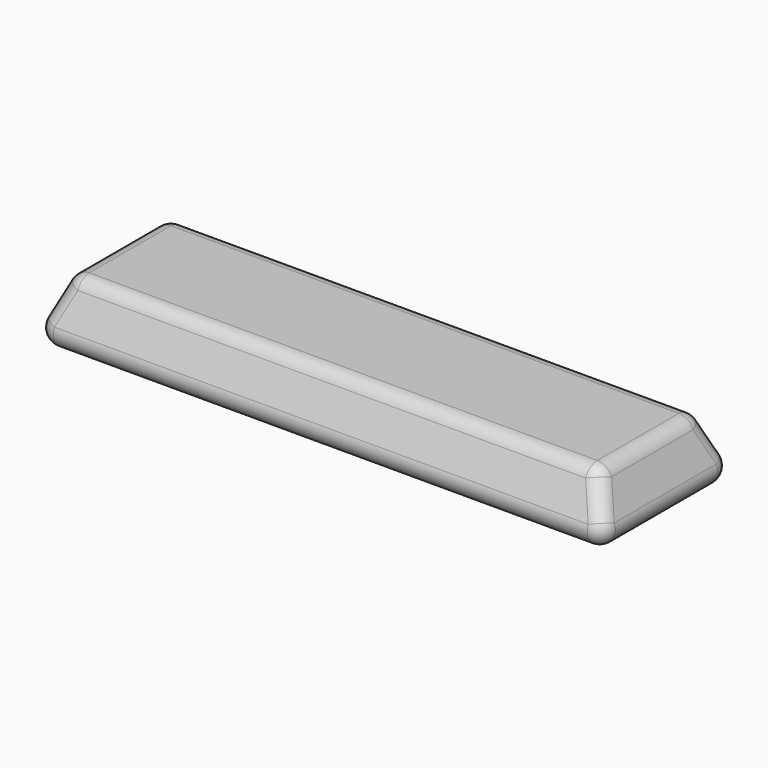
from build123d import *

# Parameters (mm, degrees)
F0_W         = 240
F0_H         = 110
F1_DEPTH     = 20
F2_T1_DEPTH  = 499.2670392907
F3_T1_DEPTH  = 865.9260025319
F4_T1_DEPTH  = 298.556361172
F5_T1_DEPTH  = 665.2153244132
F6_R         = 5
F7_T1_DEPTH  = 170.8918067496
F7_T3_DEPTH  = 40.8918067496
F7_S7_W      = 28.0904022212
F7_S7_H      = 28.0904022212
F7_T8_DEPTH  = 14.0452011106
F7_S19_W     = 28.0904022212
F7_S19_H     = 28.0904022211
F7_T20_DEPTH = 14.0452011106
F7_S31_W     = 28.0904022212
F7_S31_H     = 28.0904022212
F7_T32_DEPTH = 14.0452011106
F7_S43_W     = 28.0904022212
F7_S43_H     = 28.0904022212
F7_T44_DEPTH = 14.0452011106


# Not quite as in the source:
# - a fillet or chamfer that OpenCascade refuses, or shapes differently, is made with other operations: its cross-section is extruded or revolved along the edge and cut away or added


with BuildPart() as f1:
    # F0 (on Top) → F1 (new body)
    with BuildSketch(Plane.XY):
        Rectangle(F0_W, F0_H)
    extrude(amount=F1_DEPTH)

    # F2: chamfer of 50 x 20.7106781187 on 1 edges, made by hand

    # F2_s2 → F2_t1 (cut)
    with BuildSketch(Plane.YZ.offset(-249.6335196453)):
        Polygon((-55, -30), (-34.2893218813, 20), (-55, 20), align=None)
    extrude(amount=F2_T1_DEPTH, mode=Mode.SUBTRACT)

    # F3: chamfer of 50 x 120.7106781187 on 1 edges, made by hand

    # F3_s2 → F3_t1 (cut)
    with BuildSketch(Plane.YZ.offset(-432.9630012659)):
        Polygon((55, -100.7106781187), (5, 20), (55, 20), align=None)
    extrude(amount=F3_T1_DEPTH, mode=Mode.SUBTRACT)

    # F4: chamfer of 50 x 20.7106781187 on 1 edges, made by hand

    # F4_s2 → F4_t1 (cut)
    with BuildSketch(Plane.XZ.offset(-134.6335196453)):
        Polygon((120, -30), (99.2893218813, 20), (120, 20), align=None)
    extrude(amount=F4_T1_DEPTH, mode=Mode.SUBTRACT)

    # F5: chamfer of 50 x 120.7106781187 on 1 edges, made by hand

    # F5_s2 → F5_t1 (cut)
    with BuildSketch(Plane.XZ.offset(-317.9630012659)):
        Polygon((-120, -100.7106781187), (-70, 20), (-120, 20), align=None)
    extrude(amount=F5_T1_DEPTH, mode=Mode.SUBTRACT)

    # F6
    f6_edges = [f1.edges().sort_by_distance(p)[0] for p in [
        (103.431458, -38.431458, 10),
        (99.289322, -14.644661, 20),
        (14.644661, -34.289322, 20),
        (-74.142136, -38.431458, 10),
        (-70, -14.644661, 20),
        (-74.142136, 9.142136, 10),
        (103.431458, 9.142136, 10),
        (14.644661, 5, 20),
    ]]
    fillet(f6_edges, radius=F6_R)

    # F7: fillet of radius 5 on 8 edges, made by hand

    # F7_s2 → F7_t1 (cut)
    with BuildSketch(Plane.YZ.offset(-70.8012424341)):
        with BuildLine():
            ThreePointArc((5.8012424341, 0), (9.9585904956, 2.2221488349), (10.4206400967, 6.9134171618))
            Line((10.4206400967, 6.9134171618), (13.2842712475, 0))
            Line((13.2842712475, 0), (5.8012424341, 0))
        make_face()
        with BuildLine():
            ThreePointArc((-35.0905643154, 0), (-39.247912377, 2.2221488349), (-39.709961978, 6.9134171618))
            Line((-39.709961978, 6.9134171618), (-42.5735931288, 0))
            Line((-42.5735931288, 0), (-35.0905643154, 0))
        make_face()
    extrude(amount=F7_T1_DEPTH, mode=Mode.SUBTRACT)

    # F7_s4 → F7_t3 (cut)
    with BuildSketch(Plane.XZ.offset(-5.8012424341)):
        with BuildLine():
            ThreePointArc((-70.8012424341, 0), (-74.9585904956, 2.2221488349), (-75.4206400967, 6.9134171618))
            Line((-75.4206400967, 6.9134171618), (-78.2842712475, 0))
            Line((-78.2842712475, 0), (-70.8012424341, 0))
        make_face()
        with BuildLine():
            ThreePointArc((100.0905643154, 0), (104.247912377, 2.2221488349), (104.709961978, 6.9134171618))
            Line((104.709961978, 6.9134171618), (107.5735931288, 0))
            Line((107.5735931288, 0), (100.0905643154, 0))
        make_face()
    extrude(amount=F7_T3_DEPTH, mode=Mode.SUBTRACT)


with BuildPart() as f7_tool6:
    # F7_s7 → F7_t8 (new body)
    with BuildSketch(Plane(origin=(-36.4895727765, 36.4895727765, -9.2670771068), x_dir=(-0.7071067812, -0.7071067812, 0), z_dir=(-0.6959735574, 0.6959735574, -0.1767529771))):
        with Locations((45.9619407771, 14.4953021034)):
            Rectangle(F7_S7_W, F7_S7_H)
    extrude(amount=F7_T8_DEPTH)

    split(bisect_by=Plane.YZ.offset(-70.8012424341), keep=Keep.BOTTOM)

    split(bisect_by=Plane(origin=(-8.2432161695, 8.2432161695, -19.900884274), x_dir=(-0.7071067812, -0.7071067812, 0), z_dir=(-0.3574067443, 0.3574067443, -0.8628562095)), keep=Keep.TOP)

    split(bisect_by=Plane.XZ.offset(-5.8012424341), keep=Keep.BOTTOM)

    split(bisect_by=Plane.XY, keep=Keep.TOP)

    split(bisect_by=Plane(origin=(0, 11.3388347648, 4.6966991411), x_dir=(1, 0, 0), z_dir=(0, -0.9238795325, -0.3826834324)), keep=Keep.TOP)

    split(bisect_by=Plane(origin=(-66.8198051534, 0, 27.6776695297), x_dir=(0, 1, 0), z_dir=(0.9238795325, 0, -0.3826834324)), keep=Keep.TOP)

    # F7_s15 → F7_t16 (revolve, cut)
    with BuildSketch(Plane(origin=(-70.8012424341, 5.8012424341, 5), x_dir=(0.6959735574, -0.6959735574, 0.1767529771), z_dir=(0.1249832287, -0.1249832287, -0.9842552439))):
        with BuildLine():
            ThreePointArc((0, -5), (5, 0), (0, 5))
            Line((0, 5), (0, -5))
        make_face()
    revolve(axis=Axis((-70.8012424341, 5.8012424341, 5), (-0.7071067812, -0.7071067812, 0)), mode=Mode.SUBTRACT)


with BuildPart() as f1_1:
    add(f1.part)

    # F7_t5: cut F7_tool6
    add(f7_tool6.part, mode=Mode.SUBTRACT)


with BuildPart() as f7_tool18:
    # F7_s19 → F7_t20 (new body)
    with BuildSketch(Plane(origin=(50.6767108596, 50.6767108597, -12.8701147019), x_dir=(-0.7071067812, 0.7071067812, 0), z_dir=(0.6959735574, 0.6959735574, -0.1767529771))):
        with Locations((-66.6726188958, 18.1559761181)):
            Rectangle(F7_S19_W, F7_S19_H)
    extrude(amount=F7_T20_DEPTH)

    split(bisect_by=Plane.YZ.offset(100.0905643154), keep=Keep.TOP)

    split(bisect_by=Plane(origin=(11.9846218714, 11.9846218714, -28.9334366618), x_dir=(-0.7071067812, 0.7071067812, 0), z_dir=(0.3574067443, 0.3574067443, -0.8628562095)), keep=Keep.TOP)

    split(bisect_by=Plane.XZ.offset(-5.8012424341), keep=Keep.BOTTOM)

    split(bisect_by=Plane.XY, keep=Keep.TOP)

    split(bisect_by=Plane(origin=(0, 11.3388347648, 4.6966991411), x_dir=(1, 0, 0), z_dir=(0, -0.9238795325, -0.3826834324)), keep=Keep.TOP)

    split(bisect_by=Plane(origin=(91.8198051533, 0, 38.033008589), x_dir=(0, 1, 0), z_dir=(-0.9238795325, 0, -0.3826834324)), keep=Keep.TOP)

    # F7_s27 → F7_t28 (revolve, cut)
    with BuildSketch(Plane(origin=(100.0905643154, 5.8012424341, 5), x_dir=(-0.6959735574, -0.6959735574, 0.1767529771), z_dir=(-0.1249832287, -0.1249832287, -0.9842552439))):
        with BuildLine():
            ThreePointArc((0, -5), (5, 0), (0, 5))
            Line((0, 5), (0, -5))
        make_face()
    revolve(axis=Axis((100.0905643154, 5.8012424341, 5), (-0.7071067812, 0.7071067812, 0)), mode=Mode.SUBTRACT)


with BuildPart() as f1_2:
    add(f1_1.part)

    # F7_t17: cut F7_tool18
    add(f7_tool18.part, mode=Mode.SUBTRACT)


with BuildPart() as f7_tool30:
    # F7_s31 → F7_t32 (new body)
    with BuildSketch(Plane(origin=(-50.6767108597, -50.6767108596, -12.8701147019), x_dir=(0.7071067812, -0.7071067812, 0), z_dir=(-0.6959735574, -0.6959735574, -0.1767529771))):
        with Locations((-25.2512626585, 18.1559761181)):
            Rectangle(F7_S31_W, F7_S31_H)
    extrude(amount=F7_T32_DEPTH)

    split(bisect_by=Plane.YZ.offset(-70.8012424341), keep=Keep.BOTTOM)

    split(bisect_by=Plane(origin=(-11.9846218714, -11.9846218714, -28.9334366618), x_dir=(0.7071067812, -0.7071067812, 0), z_dir=(-0.3574067443, -0.3574067443, -0.8628562095)), keep=Keep.TOP)

    split(bisect_by=Plane.XZ.offset(35.0905643154), keep=Keep.TOP)

    split(bisect_by=Plane.XY, keep=Keep.TOP)

    split(bisect_by=Plane(origin=(0, -36.3388347648, 15.0520382004), x_dir=(1, 0, 0), z_dir=(0, 0.9238795325, -0.3826834324)), keep=Keep.TOP)

    split(bisect_by=Plane(origin=(-66.8198051534, 0, 27.6776695297), x_dir=(0, 1, 0), z_dir=(0.9238795325, 0, -0.3826834324)), keep=Keep.TOP)

    # F7_s39 → F7_t40 (revolve, cut)
    with BuildSketch(Plane(origin=(-70.8012424341, -35.0905643154, 5), x_dir=(0.6959735574, 0.6959735574, 0.1767529771), z_dir=(0.1249832287, 0.1249832287, -0.9842552439))):
        with BuildLine():
            ThreePointArc((0, -5), (5, 0), (0, 5))
            Line((0, 5), (0, -5))
        make_face()
    revolve(axis=Axis((-70.8012424341, -35.0905643154, 5), (0.7071067812, -0.7071067812, 0)), mode=Mode.SUBTRACT)


with BuildPart() as f1_3:
    add(f1_2.part)

    # F7_t29: cut F7_tool30
    add(f7_tool30.part, mode=Mode.SUBTRACT)


with BuildPart() as f7_tool42:
    # F7_s43 → F7_t44 (new body)
    with BuildSketch(Plane(origin=(64.8638489428, -64.8638489428, -16.4731522969), x_dir=(0.7071067812, 0.7071067812, 0), z_dir=(0.6959735574, -0.6959735574, -0.1767529771))):
        with Locations((45.9619407771, 21.8166501327)):
            Rectangle(F7_S43_W, F7_S43_H)
    extrude(amount=F7_T44_DEPTH)

    split(bisect_by=Plane.YZ.offset(100.0905643154), keep=Keep.TOP)

    split(bisect_by=Plane(origin=(15.7260275733, -15.7260275733, -37.9659890497), x_dir=(0.7071067812, 0.7071067812, 0), z_dir=(0.3574067443, -0.3574067443, -0.8628562095)), keep=Keep.TOP)

    split(bisect_by=Plane.XZ.offset(35.0905643154), keep=Keep.TOP)

    split(bisect_by=Plane.XY, keep=Keep.TOP)

    split(bisect_by=Plane(origin=(0, -36.3388347648, 15.0520382004), x_dir=(1, 0, 0), z_dir=(0, 0.9238795325, -0.3826834324)), keep=Keep.TOP)

    split(bisect_by=Plane(origin=(91.8198051533, 0, 38.033008589), x_dir=(0, 1, 0), z_dir=(-0.9238795325, 0, -0.3826834324)), keep=Keep.TOP)

    # F7_s51 → F7_t52 (revolve, cut)
    with BuildSketch(Plane(origin=(100.0905643154, -35.0905643154, 5), x_dir=(-0.6959735574, 0.6959735574, 0.1767529771), z_dir=(-0.1249832287, 0.1249832287, -0.9842552439))):
        with BuildLine():
            ThreePointArc((0, -5), (5, 0), (0, 5))
            Line((0, 5), (0, -5))
        make_face()
    revolve(axis=Axis((100.0905643154, -35.0905643154, 5), (0.7071067812, 0.7071067812, 0)), mode=Mode.SUBTRACT)


with BuildPart() as f1_4:
    add(f1_3.part)

    # F7_t41: cut F7_tool42
    add(f7_tool42.part, mode=Mode.SUBTRACT)


solid = f1_4.part
